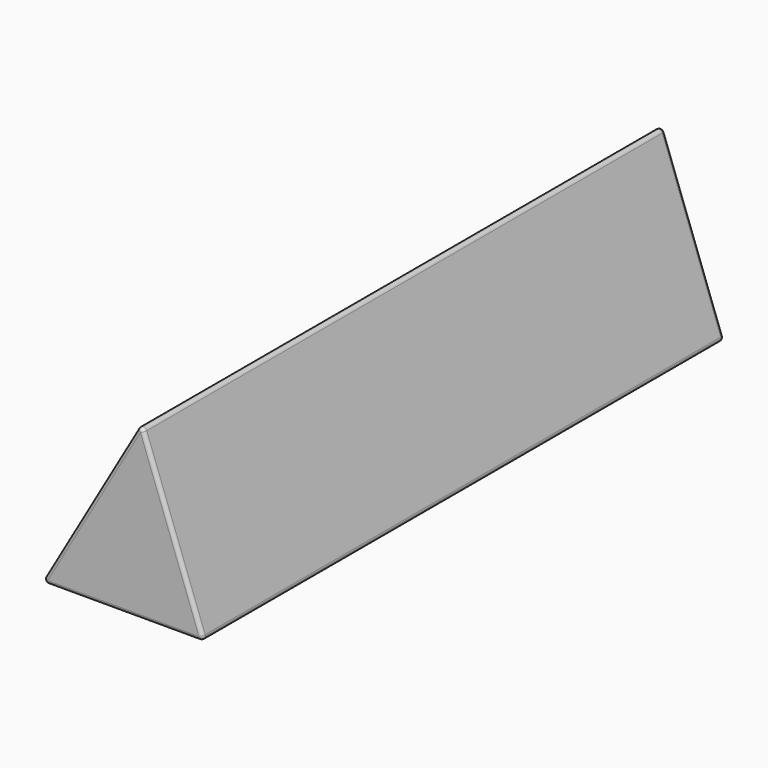
from build123d import *

# Parameters (mm, degrees)
F1_DEPTH     = 180
F2_R         = 1
F3_TEXT_SIZE = 49.7515964717
F4_DEPTH     = 2


# Not quite as in the source:
# - Text() gives the source's letters only with a copy of the font that has no kerning and outlines rounded to 1/6400 em; it was checked with that copy


with BuildPart() as f1:
    # F0 (on Front) → F1 (new body)
    with BuildSketch(Plane.XZ):
        Polygon((0, 47.7004610002), (-27.5398739989, 0), (17.3615479649, 0), align=None)
    extrude(amount=F1_DEPTH)

    # F2
    f2_edges = [f1.edges().sort_by_distance(p)[0] for p in [
        (0, -90, 47.700461),
        (-13.769937, -180, 23.850231),
        (-5.089163, -180, 0),
        (8.680774, -180, 23.850231),
        (17.361548, -90, 0),
        (-27.539874, -90, 0),
        (-13.769937, 0, 23.850231),
        (-5.089163, 0, 0),
        (8.680774, 0, 23.850231),
    ]]
    fillet(f2_edges, radius=F2_R)

    # F3 (on face) → F4 (cut)
    with BuildSketch(Plane(origin=(-20.6549054992, 0, 11.9251152501), x_dir=(0, -1, 0), z_dir=(-0.8660254038, 0, 0.5))):
        with Locations((27.7871833495, -6.1746772277)):
            Text('iHold', F3_TEXT_SIZE, font='Open Sans', font_style=FontStyle.BOLDITALIC, text_align=(TextAlign.LEFT, TextAlign.BOTTOM))
    extrude(amount=-F4_DEPTH, mode=Mode.SUBTRACT)


solid = f1.part
